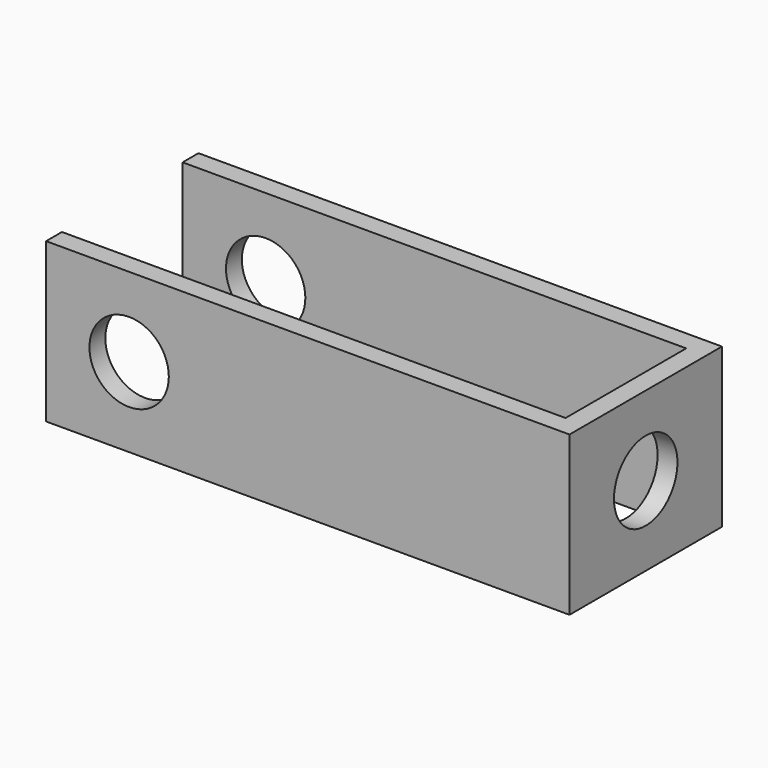
from build123d import *

# Parameters (mm, degrees)
F0_W     = 40.2857027948
F0_H     = 12.7
F0_R     = 3.175
F1_DEPTH = 1.5875
F0_W_2   = 1.5875
F2_DEPTH = 7.62
F4_R     = 3.175
F5_DEPTH = 25.4


# Not quite as in the source:
# - a length typed as a fraction of an inch, garbled in the dataset ("3 / 203.2 mm" for 3/8 in), is restored


with BuildPart() as f1:
    # F0 (on Front) → F1 (new body)
    with BuildSketch(Plane.XZ):
        with Locations((-20.1428513974, 0)):
            Rectangle(F0_W, F0_H)
        with Locations((-33.6422286928, 0)):
            Circle(F0_R, mode=Mode.SUBTRACT)
    extrude(amount=F1_DEPTH)

    # F0 (on Front) → F2 (join)
    with BuildSketch(Plane.XZ):
        with Locations((0.79375, 0)):
            Rectangle(F0_W_2, F0_H)
    extrude(amount=F2_DEPTH)

    # F3: F1 across face


with BuildPart() as f1_1:
    add(f1.part)
    add(f1.part.mirror(Plane(origin=(0.79375, -7.62, 0), x_dir=(1, 0, 0), z_dir=(0, -1, 0))))

    # F4 (on face) → F5 (cut)
    with BuildSketch(Plane(origin=(0, 0, 0), x_dir=(0, -1, 0), z_dir=(-1, 0, 0))):
        with Locations((7.62, 0)):
            Circle(F4_R)
    extrude(amount=-F5_DEPTH, mode=Mode.SUBTRACT)


solid = f1_1.part
